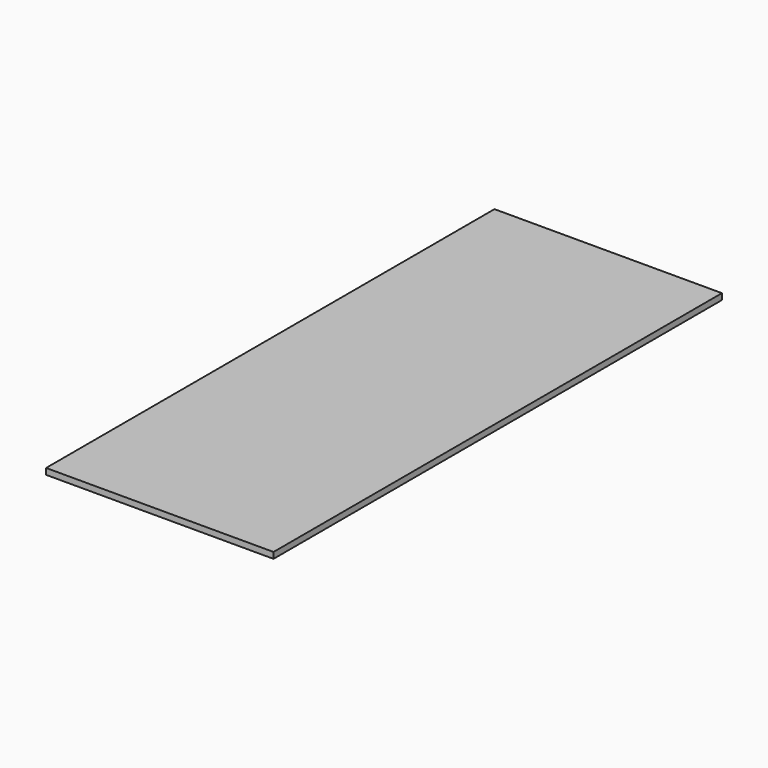
from build123d import *

# Parameters (mm, degrees)
F0_W     = 355.6
F0_H     = 876.3
F1_DEPTH = 9.525


# Not quite as in the source:
# - a length typed as a fraction of an inch, garbled in the dataset ("3 / 203.2 mm" for 3/8 in), is restored


with BuildPart() as f1:
    # F0 (on Top) → F1 (new body)
    with BuildSketch(Plane.XY):
        with Locations((177.8, 438.15)):
            Rectangle(F0_W, F0_H)
    extrude(amount=F1_DEPTH)


solid = f1.part
